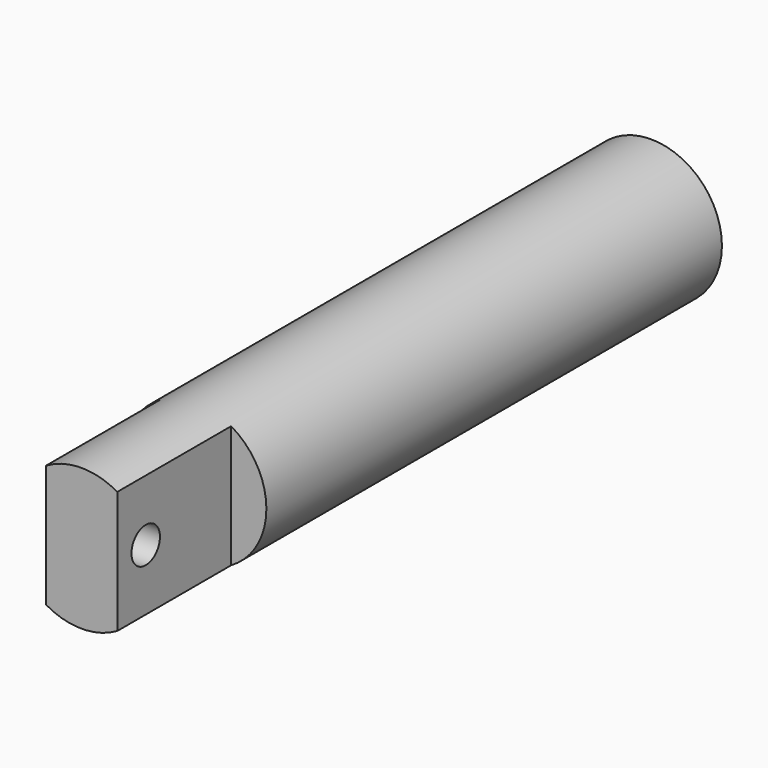
from build123d import *
from build123d import SkipClean  # not in build123d's __all__

# Parameters (mm, degrees)
F0_R     = 0.4975
F1_DEPTH = 5
F2_W     = 0.6950388919
F2_H     = 1.663880872
F3_DEPTH = 1
F4_W     = 0.4926979624
F4_H     = 1.4145199916
F5_DEPTH = 1
F6_R     = 0.125
F7_DEPTH = 25


with BuildPart() as f1:
    # F0 (on Front) → F1 (new body)
    with BuildSketch(Plane.XZ):
        Circle(F0_R)
    extrude(amount=F1_DEPTH)

    # F2 (on face) → F3 (cut)
    with BuildSketch(Plane.XZ.offset(5)):
        with Locations((-0.5975194459, 0.0155332382)):
            Rectangle(F2_W, F2_H)
    extrude(amount=-F3_DEPTH, mode=Mode.SUBTRACT)

    # F4 (on face) → F5 (cut)
    with BuildSketch(Plane.XZ.offset(5)):
        with Locations((0.4963489812, -0.1099880319)):
            Rectangle(F4_W, F4_H)
    extrude(amount=-F5_DEPTH, mode=Mode.SUBTRACT)

    # F6 (on face) → F7 (cut)
    with BuildSketch(Plane.YZ.offset(0.25)):
        with Locations((-4.75, 0)):
            Circle(F6_R)
    extrude(amount=-F7_DEPTH, mode=Mode.SUBTRACT)

    # F8 (on Right) → F9 (revolve, cut)
    with BuildSketch(Plane.YZ):
        with BuildLine():
            Line((0.25, -0.5), (0.25, 0.5))
            ThreePointArc((0.25, 0.5), (-0.25, 0), (0.25, -0.5))
        make_face()
    with SkipClean():  # cleaning this boolean's faces spoils the solid; the shape is the same uncleaned
        revolve(axis=Axis((0, 0.25, 0), (0, 0, 1)), mode=Mode.SUBTRACT)


solid = f1.part
